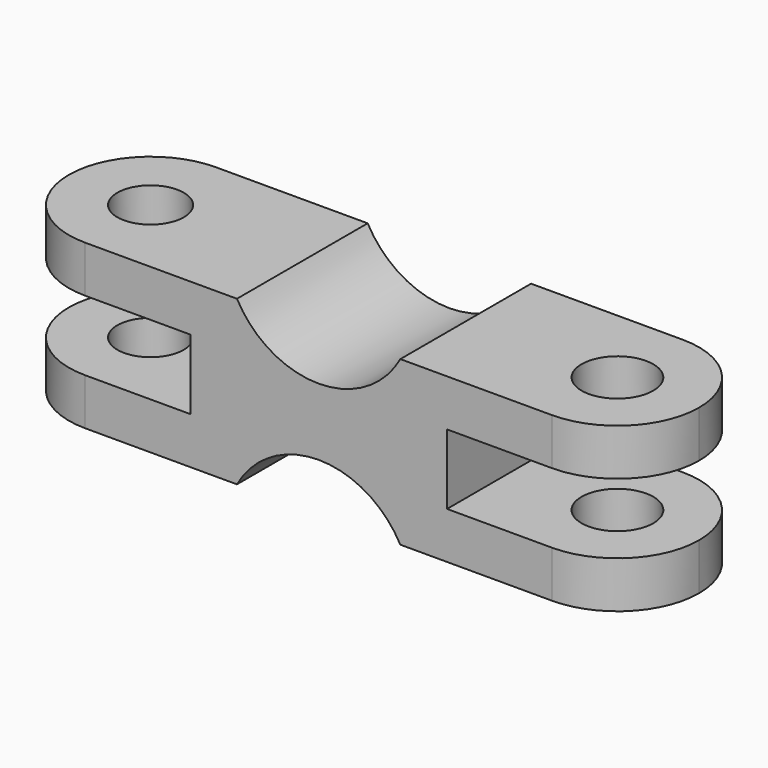
from build123d import *

# Parameters (mm, degrees)
F1_DEPTH = 5.55625
F2_R     = 1.1303
F2_R_2   = 1.2192
F3_DEPTH = 25.4
F4_R     = 2.778115


# Not quite as in the source:
# - a fillet or chamfer is up to 0.001 mm smaller than in the source, because OpenCascade refuses the exact size


with BuildPart() as f1:
    # F0 (on Front) → F1 (new body)
    with BuildSketch(Plane.XZ):
        Polygon((27.4460728326, 28.3541232628), (19.5085728326, 28.3541232628), (19.5085728326, 26.7666232628), (25.8585728326, 26.7666232628), (25.8585728326, 24.3853732628), (19.5085728326, 24.3853732628), (19.5085728326, 22.7978732628), (27.4460728326, 22.7978732628), align=None)
        with BuildLine():
            ThreePointArc((33.0023228326, 28.3541232628), (30.2241978326, 26.7162135284), (27.4460728326, 28.3541232628))
            Line((27.4460728326, 28.3541232628), (27.4460728326, 22.7978732628))
            ThreePointArc((27.4460728326, 22.7978732628), (30.2241978326, 24.4357829973), (33.0023228326, 22.7978732628))
            Line((33.0023228326, 22.7978732628), (33.0023228326, 28.3541232628))
        make_face()
        Polygon((40.9398228326, 28.3541232628), (33.0023228326, 28.3541232628), (33.0023228326, 22.7978732628), (40.9398228326, 22.7978732628), (40.9398228326, 24.3853732628), (34.5898228326, 24.3853732628), (34.5898228326, 26.7666232628), (40.9398228326, 26.7666232628), align=None)
    extrude(amount=F1_DEPTH)

    # F2 (on face) → F3 (cut)
    with BuildSketch(Plane.XY.offset(28.3541232628)):
        with Locations((22.2866978326, -2.778125)):
            Circle(F2_R)
        with Locations((38.1616978326, -2.778125)):
            Circle(F2_R_2)
    extrude(amount=-F3_DEPTH, mode=Mode.SUBTRACT)

    # F4 (radius 2.778125 in the source; OpenCascade refuses exactly that, so slightly less here)
    f4_edges = [f1.edges().sort_by_distance(p)[0] for p in [
        (19.508573, 0, 23.591623),
        (19.508573, 0, 27.560373),
        (19.508573, -5.55625, 27.560373),
        (19.508573, -5.55625, 23.591623),
        (40.939823, 0, 23.591623),
        (40.939823, 0, 27.560373),
        (40.939823, -5.55625, 23.591623),
        (40.939823, -5.55625, 27.560373),
    ]]
    fillet(f4_edges, radius=F4_R)


solid = f1.part
